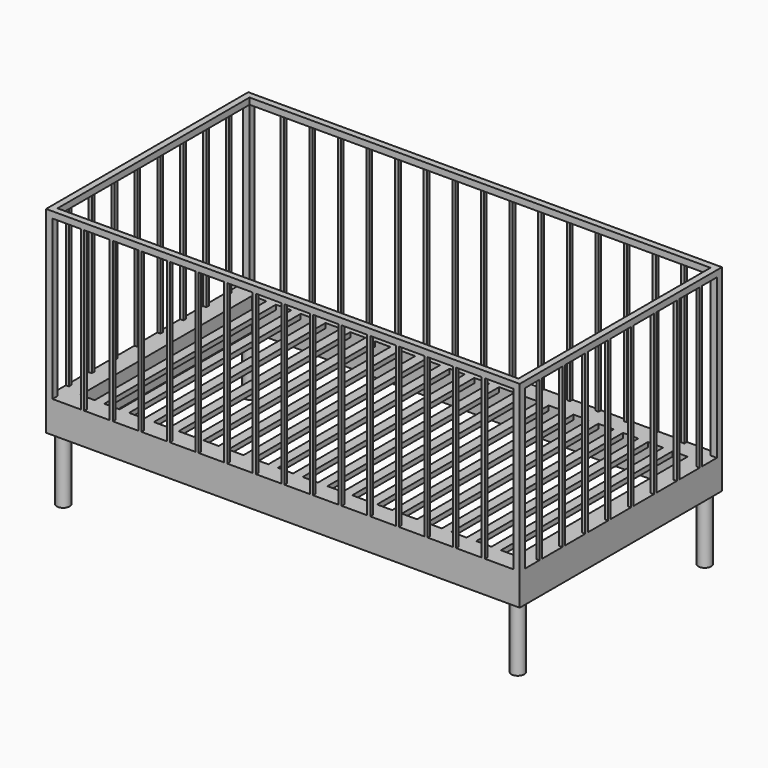
from build123d import *

# Parameters (mm, degrees)
F0_W     = 1490
F0_H     = 795
F0_W_2   = 30
F0_H_2   = 675
F1_DEPTH = 15
F2_DEPTH = 100
F3_R     = 20
F4_DEPTH = 200
F5_W     = 20
F5_H     = 20
F5_W_2   = 10
F5_H_2   = 10
F6_DEPTH = 500
F7_W     = 1450
F7_H     = 755
F8_DEPTH = 20


# Not quite as in the source:
# - a feature names something its author has since deleted; it is built from what else it names


with BuildPart() as f1:
    # F0 (on Top) → F1 (new body)
    with BuildSketch(Plane.XY):
        Rectangle(F0_W, F0_H)
        Polygon((-685, -337.5), (-685, 337.5), (-640, 337.5), (-610, 337.5), (-562, 337.5), (-532, 337.5), (-484, 337.5), (-454, 337.5), (-406, 337.5), (-376, 337.5), (-328, 337.5), (-298, 337.5), (-250, 337.5), (-220, 337.5), (-172, 337.5), (-142, 337.5), (-94, 337.5), (-64, 337.5), (-16, 337.5), (14, 337.5), (62, 337.5), (92, 337.5), (140, 337.5), (170, 337.5), (218, 337.5), (248, 337.5), (296, 337.5), (326, 337.5), (374, 337.5), (404, 337.5), (452, 337.5), (482, 337.5), (530, 337.5), (560, 337.5), (608, 337.5), (638, 337.5), (685, 337.5), (685, -337.5), (638, -337.5), (608, -337.5), (560, -337.5), (530, -337.5), (482, -337.5), (452, -337.5), (404, -337.5), (374, -337.5), (326, -337.5), (296, -337.5), (248, -337.5), (218, -337.5), (170, -337.5), (140, -337.5), (92, -337.5), (62, -337.5), (14, -337.5), (-16, -337.5), (-64, -337.5), (-94, -337.5), (-142, -337.5), (-172, -337.5), (-220, -337.5), (-250, -337.5), (-298, -337.5), (-328, -337.5), (-376, -337.5), (-406, -337.5), (-454, -337.5), (-484, -337.5), (-532, -337.5), (-562, -337.5), (-610, -337.5), (-640, -337.5), align=None, mode=Mode.SUBTRACT)
        with Locations((-625, 0)):
            Rectangle(F0_W_2, F0_H_2)
        with Locations((-547, 0)):
            Rectangle(F0_W_2, F0_H_2)
        with Locations((-469, 0)):
            Rectangle(F0_W_2, F0_H_2)
        with Locations((-391, 0)):
            Rectangle(F0_W_2, F0_H_2)
        with Locations((-313, 0)):
            Rectangle(F0_W_2, F0_H_2)
        with Locations((-235, 0)):
            Rectangle(F0_W_2, F0_H_2)
        with Locations((-157, 0)):
            Rectangle(F0_W_2, F0_H_2)
        with Locations((-79, 0)):
            Rectangle(F0_W_2, F0_H_2)
        with Locations((-1, 0)):
            Rectangle(F0_W_2, F0_H_2)
        with Locations((77, 0)):
            Rectangle(F0_W_2, F0_H_2)
        with Locations((155, 0)):
            Rectangle(F0_W_2, F0_H_2)
        with Locations((233, 0)):
            Rectangle(F0_W_2, F0_H_2)
        with Locations((311, 0)):
            Rectangle(F0_W_2, F0_H_2)
        with Locations((389, 0)):
            Rectangle(F0_W_2, F0_H_2)
        with Locations((467, 0)):
            Rectangle(F0_W_2, F0_H_2)
        with Locations((545, 0)):
            Rectangle(F0_W_2, F0_H_2)
        with Locations((623, 0)):
            Rectangle(F0_W_2, F0_H_2)
    extrude(amount=-F1_DEPTH)

    # F0 (on Top) → F2 (join)
    with BuildSketch(Plane.XY):
        Rectangle(F0_W, F0_H)
        Polygon((-685, -337.5), (-685, 337.5), (-640, 337.5), (-610, 337.5), (-562, 337.5), (-532, 337.5), (-484, 337.5), (-454, 337.5), (-406, 337.5), (-376, 337.5), (-328, 337.5), (-298, 337.5), (-250, 337.5), (-220, 337.5), (-172, 337.5), (-142, 337.5), (-94, 337.5), (-64, 337.5), (-16, 337.5), (14, 337.5), (62, 337.5), (92, 337.5), (140, 337.5), (170, 337.5), (218, 337.5), (248, 337.5), (296, 337.5), (326, 337.5), (374, 337.5), (404, 337.5), (452, 337.5), (482, 337.5), (530, 337.5), (560, 337.5), (608, 337.5), (638, 337.5), (685, 337.5), (685, -337.5), (638, -337.5), (608, -337.5), (560, -337.5), (530, -337.5), (482, -337.5), (452, -337.5), (404, -337.5), (374, -337.5), (326, -337.5), (296, -337.5), (248, -337.5), (218, -337.5), (170, -337.5), (140, -337.5), (92, -337.5), (62, -337.5), (14, -337.5), (-16, -337.5), (-64, -337.5), (-94, -337.5), (-142, -337.5), (-172, -337.5), (-220, -337.5), (-250, -337.5), (-298, -337.5), (-328, -337.5), (-376, -337.5), (-406, -337.5), (-454, -337.5), (-484, -337.5), (-532, -337.5), (-562, -337.5), (-610, -337.5), (-640, -337.5), align=None, mode=Mode.SUBTRACT)
    extrude(amount=-F2_DEPTH)

    # F3 (on face) → F4 (join)
    with BuildSketch(Plane(origin=(0, 0, -100), x_dir=(1, 0, 0), z_dir=(0, 0, -1))):
        with Locations((-715, 367.5)):
            Circle(F3_R)
        with Locations((715, 367.5)):
            Circle(F3_R)
        with Locations((715, -367.5)):
            Circle(F3_R)
        with Locations((-715, -367.5)):
            Circle(F3_R)
    extrude(amount=F4_DEPTH)

    # F5 (on face) → F6 (join)
    with BuildSketch(Plane.XY):
        with Locations((-735, 387.5)):
            Rectangle(F5_W, F5_H)
        with Locations((735, 387.5)):
            Rectangle(F5_W, F5_H)
        with Locations((-630, 392.5)):
            Rectangle(F5_W_2, F5_H_2)
        with Locations((-540, 392.5)):
            Rectangle(F5_W_2, F5_H_2)
        with Locations((-450, 392.5)):
            Rectangle(F5_W_2, F5_H_2)
        with Locations((-360, 392.5)):
            Rectangle(F5_W_2, F5_H_2)
        with Locations((-270, 392.5)):
            Rectangle(F5_W_2, F5_H_2)
        with Locations((-180, 392.5)):
            Rectangle(F5_W_2, F5_H_2)
        with Locations((-90, 392.5)):
            Rectangle(F5_W_2, F5_H_2)
        with Locations((0, 392.5)):
            Rectangle(F5_W_2, F5_H_2)
        with Locations((90, 392.5)):
            Rectangle(F5_W_2, F5_H_2)
        with Locations((180, 392.5)):
            Rectangle(F5_W_2, F5_H_2)
        with Locations((270, 392.5)):
            Rectangle(F5_W_2, F5_H_2)
        with Locations((360, 392.5)):
            Rectangle(F5_W_2, F5_H_2)
        with Locations((450, 392.5)):
            Rectangle(F5_W_2, F5_H_2)
        with Locations((540, 392.5)):
            Rectangle(F5_W_2, F5_H_2)
        with Locations((630, 392.5)):
            Rectangle(F5_W_2, F5_H_2)
        with Locations((-630, -392.5)):
            Rectangle(F5_W_2, F5_H_2)
        with Locations((-540, -392.5)):
            Rectangle(F5_W_2, F5_H_2)
        with Locations((630, -392.5)):
            Rectangle(F5_W_2, F5_H_2)
        with Locations((-735, -387.5)):
            Rectangle(F5_W, F5_H)
        with Locations((90, -392.5)):
            Rectangle(F5_W_2, F5_H_2)
        with Locations((540, -392.5)):
            Rectangle(F5_W_2, F5_H_2)
        with Locations((-450, -392.5)):
            Rectangle(F5_W_2, F5_H_2)
        with Locations((180, -392.5)):
            Rectangle(F5_W_2, F5_H_2)
        with Locations((735, -387.5)):
            Rectangle(F5_W, F5_H)
        with Locations((-360, -392.5)):
            Rectangle(F5_W_2, F5_H_2)
        with Locations((0, -392.5)):
            Rectangle(F5_W_2, F5_H_2)
        with Locations((-180, -392.5)):
            Rectangle(F5_W_2, F5_H_2)
        with Locations((360, -392.5)):
            Rectangle(F5_W_2, F5_H_2)
        with Locations((-270, -392.5)):
            Rectangle(F5_W_2, F5_H_2)
        with Locations((-90, -392.5)):
            Rectangle(F5_W_2, F5_H_2)
        with Locations((270, -392.5)):
            Rectangle(F5_W_2, F5_H_2)
        with Locations((450, -392.5)):
            Rectangle(F5_W_2, F5_H_2)
        with Locations((-740, 315)):
            Rectangle(F5_W_2, F5_H_2)
        with Locations((-740, 225)):
            Rectangle(F5_W_2, F5_H_2)
        with Locations((-740, 135)):
            Rectangle(F5_W_2, F5_H_2)
        with Locations((-740, 45)):
            Rectangle(F5_W_2, F5_H_2)
        with Locations((-740, -45)):
            Rectangle(F5_W_2, F5_H_2)
        with Locations((-740, -135)):
            Rectangle(F5_W_2, F5_H_2)
        with Locations((-740, -225)):
            Rectangle(F5_W_2, F5_H_2)
        with Locations((-740, -315)):
            Rectangle(F5_W_2, F5_H_2)
        with Locations((740, 315)):
            Rectangle(F5_W_2, F5_H_2)
        with Locations((740, 225)):
            Rectangle(F5_W_2, F5_H_2)
        with Locations((740, -135)):
            Rectangle(F5_W_2, F5_H_2)
        with Locations((740, -225)):
            Rectangle(F5_W_2, F5_H_2)
        with Locations((740, -315)):
            Rectangle(F5_W_2, F5_H_2)
        with Locations((740, 45)):
            Rectangle(F5_W_2, F5_H_2)
        with Locations((740, 135)):
            Rectangle(F5_W_2, F5_H_2)
        with Locations((740, -45)):
            Rectangle(F5_W_2, F5_H_2)
    extrude(amount=F6_DEPTH)

    # F7 (on face) → F8 (join)
    with BuildSketch(Plane.XY.offset(500)):
        Polygon((-725, 397.5), (-745, 397.5), (-745, 377.5), (-745, -397.5), (-725, -397.5), (745, -397.5), (745, 377.5), (745, 397.5), align=None)
        Rectangle(F7_W, F7_H, mode=Mode.SUBTRACT)
    extrude(amount=F8_DEPTH)


solid = f1.part
